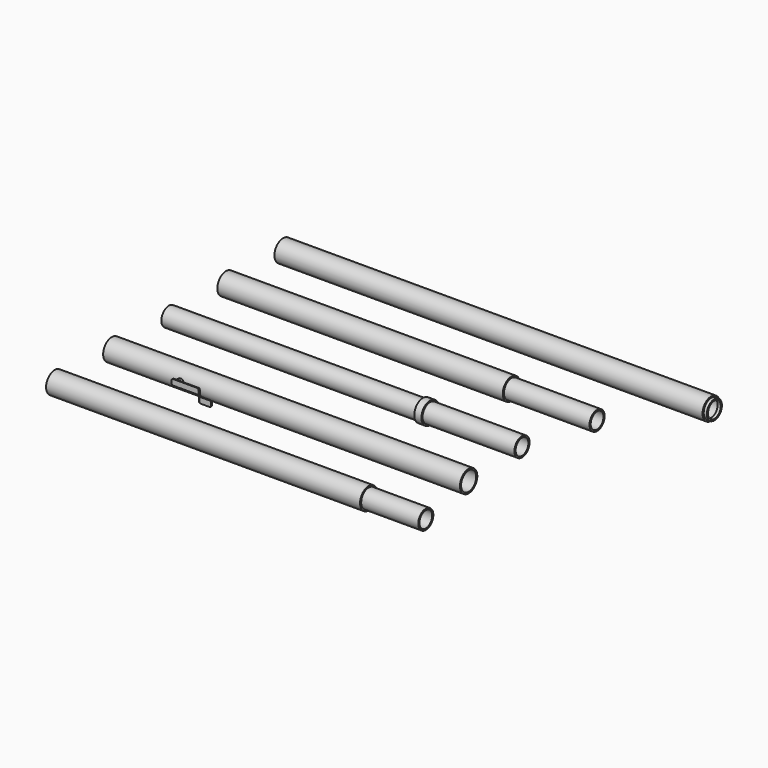
from build123d import *

# Parameters (mm, degrees)
F0_R      = 38
F0_R_2    = 32.9999953508
F1_DEPTH  = 1100
F2_R      = 32.9999953508
F2_R_2    = 28.0000001192
F3_DEPTH  = 200
F0_R_3    = 33.0000013113
F4_DEPTH  = 1250
F0_R_4    = 32.9999998212
F0_R_5    = 27.9999990016
F5_DEPTH  = 890
F6_R      = 37.9999998212
F6_R_2    = 32.9999998212
F7_DEPTH  = 25
F8_DEPTH  = 347
F0_R_6    = 32.9999983311
F9_DEPTH  = 1000
F10_R     = 32.9999983311
F10_R_2   = 27.9999956489
F11_DEPTH = 300
F0_R_7    = 33.0000042915
F12_DEPTH = 1500
F13_R     = 33.0000042915
F13_R_2   = 28.0000090599
F14_DEPTH = 11
F16_R     = 12.5
F17_DEPTH = 45
F20_DEPTH = 10
F21_R     = 5
F22_R     = 10


# Not quite as in the source:
# - the program builds the solid bodies; features that only make, move or delete a surface that nothing else refers to are left out


with BuildPart() as f1:
    # F0 (on Right) → F1 (new body)
    with BuildSketch(Plane.YZ):
        with Locations((-500, 0)):
            Circle(F0_R)
        with Locations((-500, 0)):
            Circle(F0_R_2, mode=Mode.SUBTRACT)
    extrude(amount=F1_DEPTH)


with BuildPart() as f3:
    # F2 (on face) → F3 (new body)
    with BuildSketch(Plane.YZ.offset(1100)):
        with Locations((-500, 0)):
            Circle(F2_R)
        with Locations((-500, 0)):
            Circle(F2_R_2, mode=Mode.SUBTRACT)
    extrude(amount=F3_DEPTH)


with BuildPart() as f4:
    # F0 (on Right) → F4 (new body)
    with BuildSketch(Plane.YZ):
        with Locations((-250, 0)):
            Circle(F0_R)
        with Locations((-250, 0)):
            Circle(F0_R_3, mode=Mode.SUBTRACT)
    extrude(amount=F4_DEPTH)


with BuildPart() as f5:
    # F0 (on Right) → F5 (new body)
    with BuildSketch(Plane.YZ):
        Circle(F0_R_4)
        Circle(F0_R_5, mode=Mode.SUBTRACT)
    extrude(amount=F5_DEPTH)


with BuildPart() as f7:
    # F6 (on face) → F7 (new body)
    with BuildSketch(Plane.YZ.offset(890)):
        Circle(F6_R)
        Circle(F6_R_2, mode=Mode.SUBTRACT)
    extrude(amount=F7_DEPTH)


with BuildPart() as f8:
    # F8 (new): a face of the model
    f8_faces = [f5.part.faces().sort_by_distance(p)[0] for p in [
        (890, -32.0666188751, 0),
    ]]
    extrude(f8_faces, amount=F8_DEPTH)


with BuildPart() as f9:
    # F0 (on Right) → F9 (new body)
    with BuildSketch(Plane.YZ):
        with Locations((250, 0)):
            Circle(F0_R)
        with Locations((250, 0)):
            Circle(F0_R_6, mode=Mode.SUBTRACT)
    extrude(amount=F9_DEPTH)


with BuildPart() as f11:
    # F10 (on face) → F11 (new body)
    with BuildSketch(Plane.YZ.offset(1000)):
        with Locations((250, 0)):
            Circle(F10_R)
        with Locations((250, 0)):
            Circle(F10_R_2, mode=Mode.SUBTRACT)
    extrude(amount=F11_DEPTH)


with BuildPart() as f12:
    # F0 (on Right) → F12 (new body)
    with BuildSketch(Plane.YZ):
        with Locations((500, 0)):
            Circle(F0_R)
        with Locations((500, 0)):
            Circle(F0_R_7, mode=Mode.SUBTRACT)
    extrude(amount=F12_DEPTH)


with BuildPart() as f14:
    # F13 (on face) → F14 (new body)
    with BuildSketch(Plane.YZ.offset(1500)):
        with Locations((500, 0)):
            Circle(F13_R)
        with Locations((500, 0)):
            Circle(F13_R_2, mode=Mode.SUBTRACT)
    extrude(amount=F14_DEPTH)


with BuildPart() as f17:
    # F16 (on plane+point) → F17 (new body)
    with BuildSketch(Plane.XZ.offset(250)):
        with Locations((270, 0)):
            Circle(F16_R)
    extrude(amount=F17_DEPTH)

    # F18 (on Top) → F20 (join, symmetric)
    with BuildSketch(Plane.XY):
        Polygon((343.6963860454, -295), (248.1320642157, -295), (248.1320642157, -298), (342.3292072788, -298), (374.479667039, -334.9848731859), (396.771981816, -334.9848731859), (400.771981816, -334.9848731859), (415.771981816, -334.9848731859), (415.771981816, -331.9848731859), (375.8468458056, -331.9848731859), align=None)
    extrude(amount=F20_DEPTH, both=True)

    # F21
    f21_edges = [f17.edges().sort_by_distance(p)[0] for p in [
        (415.771982, -333.484873, 10),
        (415.771982, -333.484873, -10),
        (248.132064, -296.5, 10),
        (248.132064, -296.5, -10),
    ]]
    fillet(f21_edges, radius=F21_R)

    # F22
    f22_edges = [f17.edges().sort_by_distance(p)[0] for p in [
        (342.329207, -298, 0),
        (374.479667, -334.984873, 0),
        (375.846846, -331.984873, 0),
        (343.696386, -295, 0),
    ]]
    fillet(f22_edges, radius=F22_R)


solid = Compound([f1.part, f3.part, f4.part, f5.part, f7.part, f8.part, f9.part, f11.part, f12.part, f14.part, f17.part])
